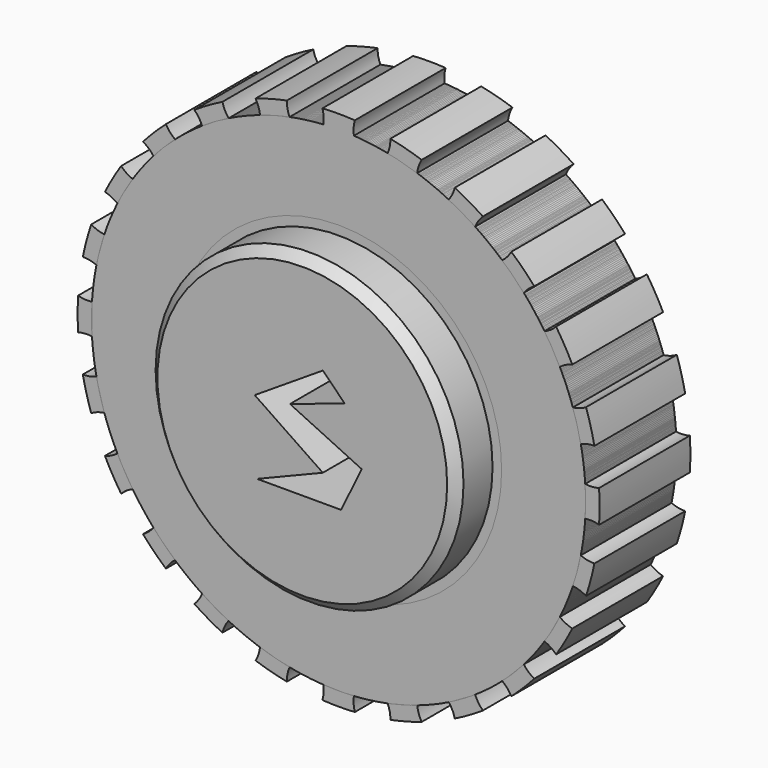
from build123d import *

# Parameters (mm, degrees)
F0_R      = 33.9209141307
F1_DEPTH  = 25
F2_COUNT  = 24
F0_R_2    = 21.7005672346
F3_DEPTH  = 35
F4_SIZE   = 2
F4_2_SIZE = 2


with BuildPart() as f1:
    # F0 (on Front) → F1 (new body)
    with BuildSketch(Plane.XZ):
        with BuildLine():
            ThreePointArc((3.3660312813, 54.335799998), (3.3044933999, 55.8752247224), (3.5729595926, 57.3923078764))
            ThreePointArc((3.5729595926, 57.3923078764), (0, 57.5034176691), (-3.5729595926, 57.3923078764))
            ThreePointArc((-3.5729595926, 57.3923078764), (-3.3044933999, 55.8752247224), (-3.3660312813, 54.335799998))
            ThreePointArc((-3.3660312813, 54.335799998), (0, 54.4399607642), (3.3660312813, 54.335799998))
        make_face()
        with BuildLine():
            ThreePointArc((54.4399607642, 0), (39.6670892484, 37.2858063955), (3.3660312813, 54.335799998))
            ThreePointArc((3.3660312813, 54.335799998), (0, 54.4399607642), (-3.3660312813, 54.335799998))
            ThreePointArc((-3.3660312813, 54.335799998), (-37.2858063955, -39.6670892484), (54.4399607642, 0))
        make_face()
        Circle(F0_R, mode=Mode.SUBTRACT)
    extrude(amount=F1_DEPTH)


with BuildPart() as f2_1:
    # F2: instance of F1
    add(f1.part.rotate(Axis((0, 0, 0), (0, -1, 0)), 1 * 360 / F2_COUNT))


with BuildPart() as f2_2:
    # F2: instance of F1
    add(f1.part.rotate(Axis((0, 0, 0), (0, -1, 0)), 2 * 360 / F2_COUNT))


with BuildPart() as f2_3:
    # F2: instance of F1
    add(f1.part.rotate(Axis((0, 0, 0), (0, -1, 0)), 3 * 360 / F2_COUNT))


with BuildPart() as f2_4:
    # F2: instance of F1
    add(f1.part.rotate(Axis((0, 0, 0), (0, -1, 0)), 4 * 360 / F2_COUNT))


with BuildPart() as f2_5:
    # F2: instance of F1
    add(f1.part.rotate(Axis((0, 0, 0), (0, -1, 0)), 5 * 360 / F2_COUNT))


with BuildPart() as f2_6:
    # F2: instance of F1
    add(f1.part.rotate(Axis((0, 0, 0), (0, -1, 0)), 6 * 360 / F2_COUNT))


with BuildPart() as f2_7:
    # F2: instance of F1
    add(f1.part.rotate(Axis((0, 0, 0), (0, -1, 0)), 7 * 360 / F2_COUNT))


with BuildPart() as f2_8:
    # F2: instance of F1
    add(f1.part.rotate(Axis((0, 0, 0), (0, -1, 0)), 8 * 360 / F2_COUNT))


with BuildPart() as f2_9:
    # F2: instance of F1
    add(f1.part.rotate(Axis((0, 0, 0), (0, -1, 0)), 9 * 360 / F2_COUNT))


with BuildPart() as f2_10:
    # F2: instance of F1
    add(f1.part.rotate(Axis((0, 0, 0), (0, -1, 0)), 10 * 360 / F2_COUNT))


with BuildPart() as f2_11:
    # F2: instance of F1
    add(f1.part.rotate(Axis((0, 0, 0), (0, -1, 0)), 11 * 360 / F2_COUNT))


with BuildPart() as f2_12:
    # F2: instance of F1
    add(f1.part.rotate(Axis((0, 0, 0), (0, -1, 0)), 12 * 360 / F2_COUNT))


with BuildPart() as f2_13:
    # F2: instance of F1
    add(f1.part.rotate(Axis((0, 0, 0), (0, -1, 0)), 13 * 360 / F2_COUNT))


with BuildPart() as f2_14:
    # F2: instance of F1
    add(f1.part.rotate(Axis((0, 0, 0), (0, -1, 0)), 14 * 360 / F2_COUNT))


with BuildPart() as f2_15:
    # F2: instance of F1
    add(f1.part.rotate(Axis((0, 0, 0), (0, -1, 0)), 15 * 360 / F2_COUNT))


with BuildPart() as f2_16:
    # F2: instance of F1
    add(f1.part.rotate(Axis((0, 0, 0), (0, -1, 0)), 16 * 360 / F2_COUNT))


with BuildPart() as f2_17:
    # F2: instance of F1
    add(f1.part.rotate(Axis((0, 0, 0), (0, -1, 0)), 17 * 360 / F2_COUNT))


with BuildPart() as f2_18:
    # F2: instance of F1
    add(f1.part.rotate(Axis((0, 0, 0), (0, -1, 0)), 18 * 360 / F2_COUNT))


with BuildPart() as f2_19:
    # F2: instance of F1
    add(f1.part.rotate(Axis((0, 0, 0), (0, -1, 0)), 19 * 360 / F2_COUNT))


with BuildPart() as f2_20:
    # F2: instance of F1
    add(f1.part.rotate(Axis((0, 0, 0), (0, -1, 0)), 20 * 360 / F2_COUNT))


with BuildPart() as f2_21:
    # F2: instance of F1
    add(f1.part.rotate(Axis((0, 0, 0), (0, -1, 0)), 21 * 360 / F2_COUNT))


with BuildPart() as f2_22:
    # F2: instance of F1
    add(f1.part.rotate(Axis((0, 0, 0), (0, -1, 0)), 22 * 360 / F2_COUNT))


with BuildPart() as f2_23:
    # F2: instance of F1
    add(f1.part.rotate(Axis((0, 0, 0), (0, -1, 0)), 23 * 360 / F2_COUNT))


with BuildPart() as f3:
    # F0 (on Front) → F3 (new body)
    with BuildSketch(Plane.XZ):
        Circle(F0_R)
        Circle(F0_R_2, mode=Mode.SUBTRACT)
        Circle(F0_R_2)
        Polygon((-10.4838311672, 3.5842789803), (4.5198369771, 13.2294967771), (9.3424450606, 8.4068877622), (-2.7140742168, 4.3880473822), (13.093367219, -3.1137887854), (8.5386764258, -12.4910827726), (-9.9479854107, -12.4910827726), (4.5198369771, -6.5967836417), align=None, mode=Mode.SUBTRACT)
    extrude(amount=F3_DEPTH)

    # F4
    f4_edges = [f3.edges().sort_by_distance(p)[0] for p in [
        (-33.920914, -35, 0),
    ]]
    chamfer(f4_edges, length=F4_SIZE)


with BuildPart() as f1_1:
    add(f1.part)

    # F4#2
    f4_2_edges = [f1_1.edges().sort_by_distance(p)[0] for p in [
        (-33.920914, -25, 0),
    ]]
    chamfer(f4_2_edges, length=F4_2_SIZE)


solid = Compound([f2_1.part, f2_2.part, f2_3.part, f2_4.part, f2_5.part, f2_6.part, f2_7.part, f2_8.part, f2_9.part, f2_10.part, f2_11.part, f2_12.part, f2_13.part, f2_14.part, f2_15.part, f2_16.part, f2_17.part, f2_18.part, f2_19.part, f2_20.part, f2_21.part, f2_22.part, f2_23.part, f3.part, f1_1.part])
